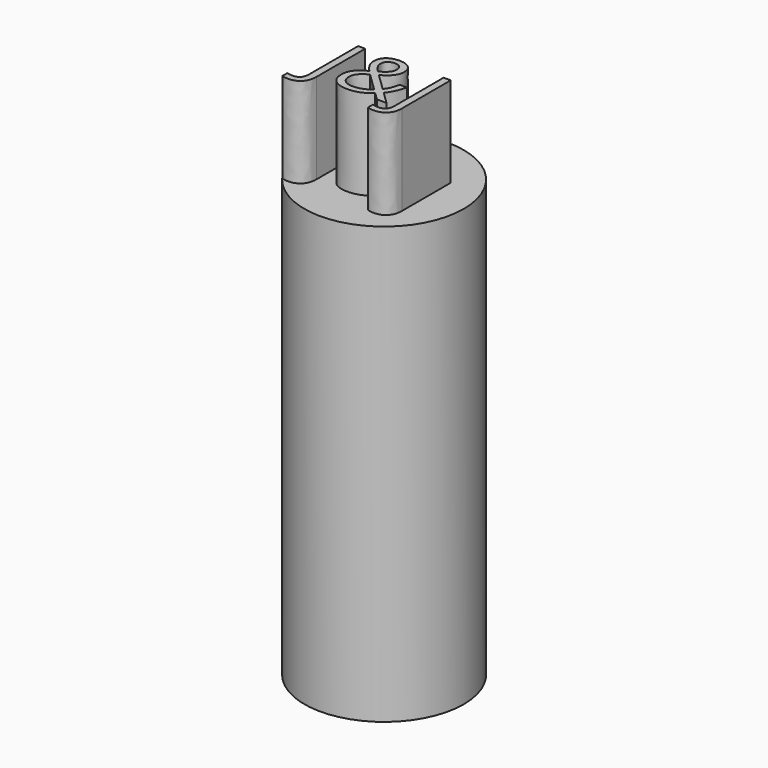
from build123d import *

# Parameters (mm, degrees)
F1_R         = 22.0710965494
F2_DEPTH     = 120.8
F0_R         = 18.9040058903
F3_DEPTH     = 25
F4_TEXT_SIZE = 23.7505818303
F5_DEPTH     = 25


# Not quite as in the source:
# - Text() gives the source's letters only with a copy of the font that has no kerning and outlines rounded to 1/6400 em; it was checked with that copy


with BuildPart() as f2:
    # F1 (on Top) → F2 (new body)
    with BuildSketch(Plane.XY):
        Circle(F1_R)
    extrude(amount=F2_DEPTH)

    # F0 (on Top) → F3 (join)
    with BuildSketch(Plane.XY):
        Circle(F0_R)
    extrude(amount=F3_DEPTH)

    # F4 (on face) → F5 (join)
    with BuildSketch(Plane.XY.offset(120.8)):
        with Locations((-15.6252851245, -9.170377627)):
            Text('J&J', F4_TEXT_SIZE, font='Open Sans', text_align=(TextAlign.LEFT, TextAlign.BOTTOM))
    extrude(amount=F5_DEPTH)


solid = f2.part
